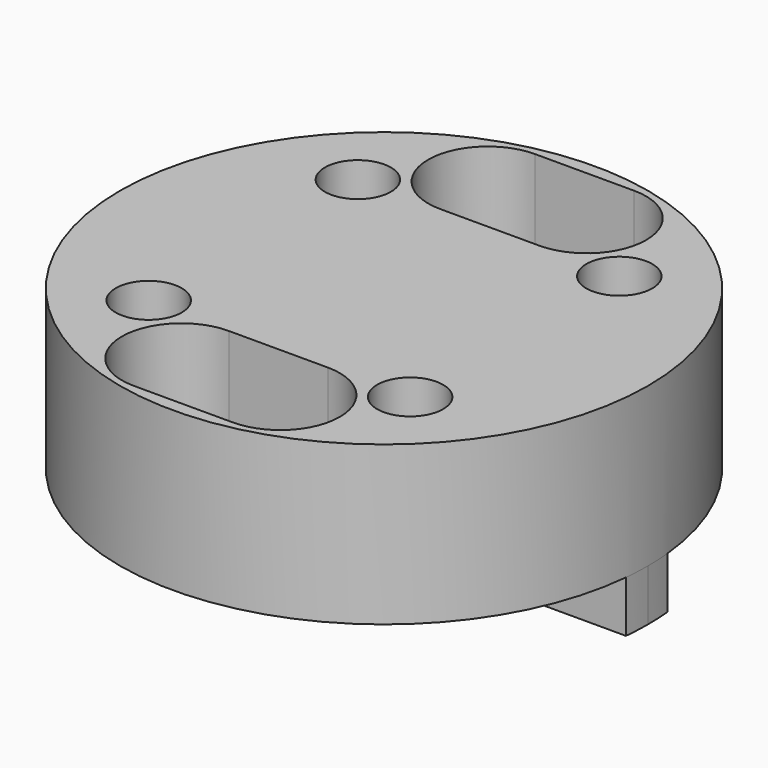
from build123d import *

# Parameters (mm, degrees)
F0_R     = 20
F0_R_2   = 2.5
F1_DEPTH = 12
F3_DEPTH = 3.9
F5_DEPTH = 15.901
F7_DEPTH = 8


# Not quite as in the source:
# - after a boolean that leaves OpenCascade's solid faulty, fix() repairs it


with BuildPart() as f1:
    # F0 (on Top) → F1 (new body)
    with BuildSketch(Plane.XY):
        Circle(F0_R)
        with Locations((-9.8994949366, -9.8994949366)):
            Circle(F0_R_2, mode=Mode.SUBTRACT)
        with Locations((9.8994949366, -9.8994949366)):
            Circle(F0_R_2, mode=Mode.SUBTRACT)
        with Locations((-9.8994949366, 9.8994949366)):
            Circle(F0_R_2, mode=Mode.SUBTRACT)
        with Locations((9.8994949366, 9.8994949366)):
            Circle(F0_R_2, mode=Mode.SUBTRACT)
    extrude(amount=F1_DEPTH)

    # F2 (on face) → F3 (join)
    with BuildSketch(Plane(origin=(0, 0, 0), x_dir=(1, 0, 0), z_dir=(0, 0, -1))):
        with BuildLine():
            Line((19.9022454763, 1.975), (-19.9022454763, 1.975))
            ThreePointArc((-19.9022454763, 1.975), (-20, 0), (-19.9022454763, -1.975))
            Line((-19.9022454763, -1.975), (19.9022454763, -1.975))
            ThreePointArc((19.9022454763, -1.975), (19.9755464196, -0.9887088736), (20, 0))
            ThreePointArc((20, 0), (19.9755464196, 0.9887088736), (19.9022454763, 1.975))
        make_face()
    extrude(amount=F3_DEPTH)

    add(f1.part.fix(), mode=Mode.REPLACE)

    # F4 (on face) → F5 (cut, through all)
    with BuildSketch(Plane.XY.offset(12)):
        with BuildLine():
            Line((3.75, 17.5), (-3.75, 17.5))
            ThreePointArc((-3.75, 17.5), (-6.75, 14.5), (-3.75, 11.5))
            Line((-3.75, 11.5), (3.75, 11.5))
            ThreePointArc((3.75, 11.5), (6.75, 14.5), (3.75, 17.5))
        make_face()
        with BuildLine():
            ThreePointArc((3.75, -17.5), (6.75, -14.5), (3.75, -11.5))
            Line((3.75, -11.5), (-3.75, -11.5))
            ThreePointArc((-3.75, -11.5), (-6.75, -14.5), (-3.75, -17.5))
            Line((-3.75, -17.5), (3.75, -17.5))
        make_face()
    extrude(amount=-F5_DEPTH, mode=Mode.SUBTRACT)

    # F6 (on face) → F7 (cut)
    with BuildSketch(Plane.XY.offset(12)):
        with BuildLine():
            Line((3.75, 19), (-3.75, 19))
            ThreePointArc((-3.75, 19), (-8.25, 14.5), (-3.75, 10))
            Line((-3.75, 10), (3.75, 10))
            ThreePointArc((3.75, 10), (8.25, 14.5), (3.75, 19))
        make_face()
        with BuildLine():
            ThreePointArc((-3.75, 11.5), (-6.75, 14.5), (-3.75, 17.5))
            Line((-3.75, 17.5), (3.75, 17.5))
            ThreePointArc((3.75, 17.5), (6.75, 14.5), (3.75, 11.5))
            Line((3.75, 11.5), (-3.75, 11.5))
        make_face(mode=Mode.SUBTRACT)
        with BuildLine():
            ThreePointArc((3.75, -19), (8.25, -14.5), (3.75, -10))
            Line((3.75, -10), (-3.75, -10))
            ThreePointArc((-3.75, -10), (-8.25, -14.5), (-3.75, -19))
            Line((-3.75, -19), (3.75, -19))
        make_face()
        with BuildLine():
            ThreePointArc((3.75, -11.5), (6.75, -14.5), (3.75, -17.5))
            Line((3.75, -17.5), (-3.75, -17.5))
            ThreePointArc((-3.75, -17.5), (-6.75, -14.5), (-3.75, -11.5))
            Line((-3.75, -11.5), (3.75, -11.5))
        make_face(mode=Mode.SUBTRACT)
    extrude(amount=-F7_DEPTH, mode=Mode.SUBTRACT)


solid = f1.part
